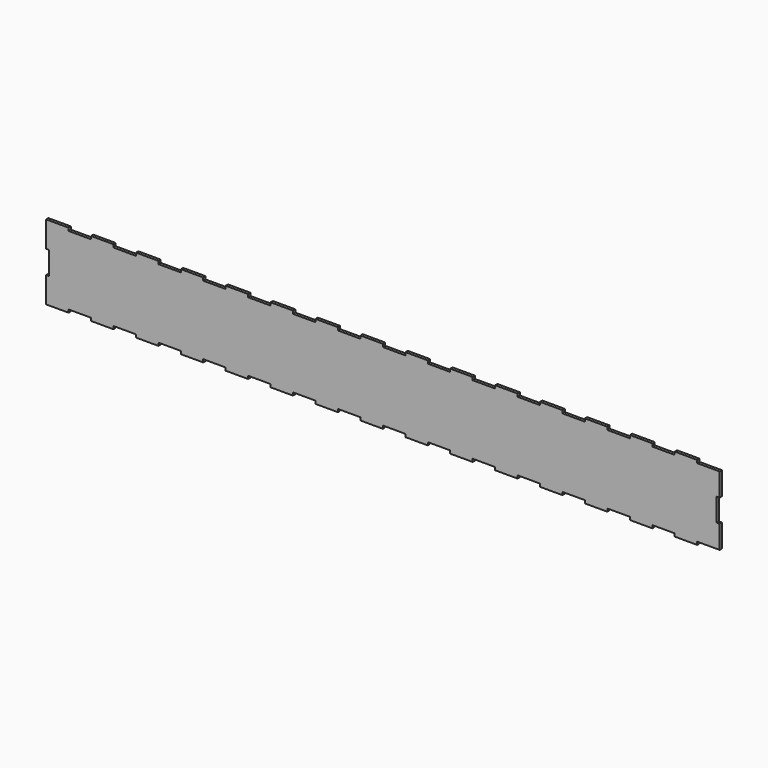
from build123d import *

# Parameters (mm, degrees)
F1_DEPTH = 3.175


# Not quite as in the source:
# - ends of sketch curves that miss each other by under 0.0002 mm in the source are joined


with BuildPart() as f1:
    # F0 (on Front) → F1 (new body)
    with BuildSketch(Plane.XZ):
        Polygon((148.5900335276, 41.2750068545), (123.8250335276, 41.2750068545), (123.8250335276, 38.1000068545), (99.0600335276, 38.1000068545), (99.0600335276, 41.2750068545), (74.2950335276, 41.2750068545), (74.2950335276, 38.1000068545), (49.5300335276, 38.1000068545), (49.5300335276, 41.2750068545), (24.7650335276, 41.2750068545), (24.7650335276, 38.1000068545), (3.35276e-05, 38.1000068545), (3.35276e-05, 41.2750068545), (-24.7649664724, 41.2750068545), (-24.7649664724, 38.1000068545), (-49.5299664724, 38.1000068545), (-49.5299664724, 41.2750068545), (-74.2949664724, 41.2750068545), (-74.2949664724, 38.1000068545), (-99.0599664724, 38.1000068545), (-99.0599664724, 41.2750068545), (-123.8249664724, 41.2750068545), (-123.8249664724, 38.1000068545), (-148.5899664724, 38.1000068545), (-148.5899664724, 41.2750068545), (-173.3549664724, 41.2750068545), (-173.3549664724, 38.1000068545), (-198.1199664724, 38.1000068545), (-198.1199664724, 41.2750068545), (-222.8849664724, 41.2750068545), (-222.8849664724, 38.1000068545), (-247.6499664724, 38.1000068545), (-247.6499664724, 41.2750068545), (-272.4149664724, 41.2750068545), (-272.4149664724, 38.1000068545), (-297.1799664724, 38.1000068545), (-297.1799664724, 41.2750068545), (-321.9449664724, 41.2750068545), (-321.9449664724, 38.1000068545), (-346.7099664724, 38.1000068545), (-346.7099664724, 41.2750068545), (-371.4749664724, 41.2750068545), (-371.475, 38.1), (-371.475, 12.7), (-368.3, 12.7), (-368.3, -12.7), (-371.475, -12.7), (-371.475, -38.1), (-371.475031665, -41.2750032454), (-346.710031665, -41.2750032454), (-346.710031665, -38.1000032454), (-321.945031665, -38.1000032454), (-321.945031665, -41.2750032454), (-297.180031665, -41.2750032454), (-297.180031665, -38.1000032454), (-272.415031665, -38.1000032454), (-272.415031665, -41.2750032454), (-247.650031665, -41.2750032454), (-247.650031665, -38.1000032454), (-222.885031665, -38.1000032454), (-222.885031665, -41.2750032454), (-198.120031665, -41.2750032454), (-198.120031665, -38.1000032454), (-173.355031665, -38.1000032454), (-173.355031665, -41.2750032454), (-148.590031665, -41.2750032454), (-148.590031665, -38.1000032454), (-123.825031665, -38.1000032454), (-123.825031665, -41.2750032454), (-99.060031665, -41.2750032454), (-99.060031665, -38.1000032454), (-74.295031665, -38.1000032454), (-74.295031665, -41.2750032454), (-49.530031665, -41.2750032454), (-49.530031665, -38.1000032454), (-24.765031665, -38.1000032454), (-24.765031665, -41.2750032454), (-3.1665e-05, -41.2750032454), (-3.1665e-05, -38.1000032454), (24.764968335, -38.1000032454), (24.764968335, -41.2750032454), (49.529968335, -41.2750032454), (49.529968335, -38.1000032454), (74.294968335, -38.1000032454), (74.294968335, -41.2750032454), (92.075, -41.2750032454), (99.059968335, -41.2750032454), (99.059968335, -38.1000032454), (123.824968335, -38.1000032454), (123.824968335, -41.2750032454), (148.589968335, -41.2750032454), (148.589968335, -38.1000032454), (173.354968335, -38.1000032454), (173.354968335, -41.2750032454), (198.119968335, -41.2750032454), (198.119968335, -38.1000032454), (222.884968335, -38.1000032454), (222.884968335, -41.2750032454), (244.475, -41.2750032454), (247.649968335, -41.2750032454), (247.649968335, -38.1000032454), (272.414968335, -38.1000032454), (272.414968335, -41.2750032454), (297.179968335, -41.2750032454), (297.179968335, -38.1000032454), (321.944968335, -38.1000032454), (321.944968335, -41.2750032454), (346.709968335, -41.2750032453), (346.709968335, -38.1000032454), (371.474968335, -38.0999963909), (371.475, -12.7), (368.3, -12.7), (368.3, 12.7), (371.475, 12.7), (371.475, 38.1), (368.3, 38.1), (346.7100335276, 38.1), (346.7100335276, 41.2750068545), (321.9450335276, 41.2750068544), (321.9450335276, 38.1000068545), (297.1800335276, 38.1000068545), (297.1800335276, 41.2750068545), (272.4150335276, 41.2750068545), (272.4150335276, 38.1000068545), (247.6500335276, 38.1000068545), (247.6500335276, 41.2750068545), (222.8850335276, 41.2750068545), (222.8850335276, 38.1000068545), (198.1200335276, 38.1000068545), (198.1200335276, 41.2750068545), (173.3550335276, 41.2750068545), (173.3550335276, 38.1000068545), (148.5900335276, 38.1000068545), align=None)
    extrude(amount=F1_DEPTH)


solid = f1.part
